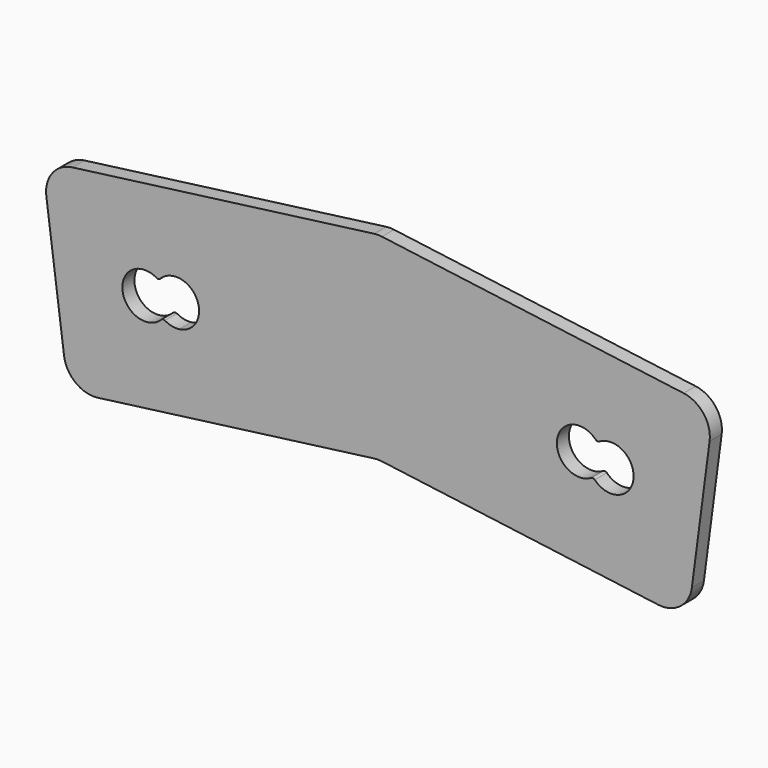
from build123d import *

# Parameters (mm, degrees)
F1_DEPTH = 3.175
F2_R     = 12.7
F3_R     = 1.27
F4_R     = 1.27


with BuildPart() as f1:
    # F0 (on Front) → F1 (new body, symmetric)
    with BuildSketch(Plane.XZ):
        Polygon((-79.404899, -10.453853), (0, 0), (0, 83.262321), (-141.215347, 64.670968), (-130.44041, -17.172806), align=None)
        with BuildLine():
            ThreePointArc((-75.267368, 30.468033), (-77.631094, 24.187764), (-83.549106, 21.024521))
            ThreePointArc((-83.549106, 21.024521), (-87.225447, 21.25903), (-90.537856, 22.870995))
            ThreePointArc((-90.537856, 22.870995), (-107.497341, 27.478867), (-92.308341, 36.319167))
            ThreePointArc((-92.308341, 36.319167), (-81.699151, 39.476787), (-75.267368, 30.468033))
        make_face(mode=Mode.SUBTRACT)
        Polygon((0, 83.262321), (0, 0), (130.44041, -17.172806), (141.215347, 64.670968), align=None)
        with BuildLine():
            ThreePointArc((90.537856, 22.870995), (75.348856, 31.711295), (92.308341, 36.319167))
            ThreePointArc((92.308341, 36.319167), (102.296461, 37.250065), (107.578829, 28.722129))
            ThreePointArc((107.578829, 28.722129), (101.147046, 19.713376), (90.537856, 22.870995))
        make_face(mode=Mode.SUBTRACT)
    extrude(amount=F1_DEPTH, both=True)

    # F2
    f2_edges = [f1.edges().sort_by_distance(p)[0] for p in [
        (-141.215347, 0, 64.670968),
        (0, 0, 83.262321),
        (0, 0, 0),
        (130.44041, 0, -17.172806),
        (141.215347, 0, 64.670968),
        (-130.44041, 0, -17.172806),
    ]]
    fillet(f2_edges, radius=F2_R)

    # F3
    f3_edges = [f1.edges().sort_by_distance(p)[0] for p in [
        (-92.308341, 0, 36.319167),
        (-90.537856, 0, 22.870995),
    ]]
    fillet(f3_edges, radius=F3_R)

    # F4
    f4_edges = [f1.edges().sort_by_distance(p)[0] for p in [
        (90.537856, 0, 22.870995),
        (92.308341, 0, 36.319167),
    ]]
    fillet(f4_edges, radius=F4_R)


solid = f1.part
